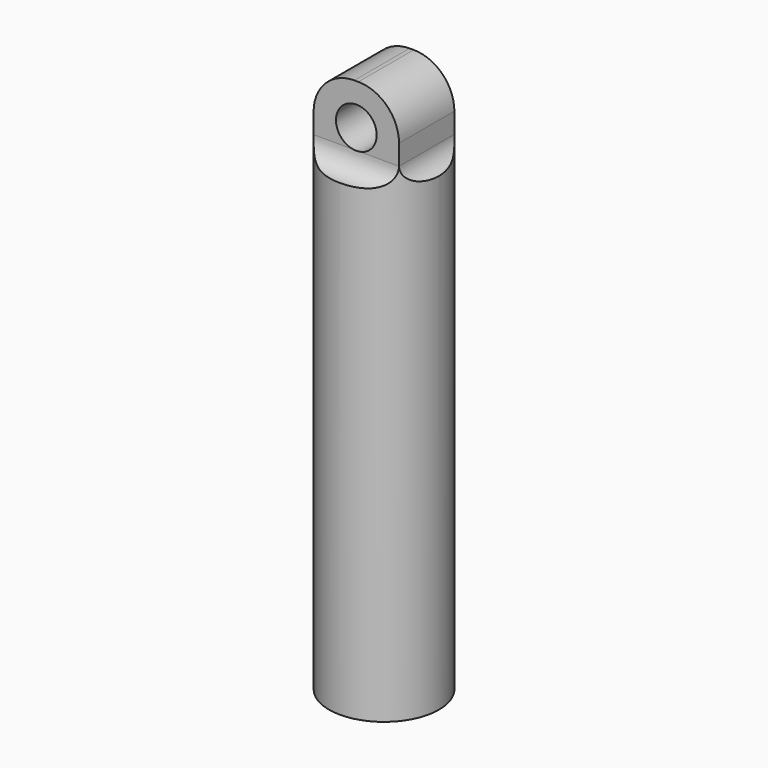
from build123d import *

# Parameters (mm, degrees)
F0_R         = 13.5
F1_DEPTH     = 115
F2_W         = 20.9761769634
F2_H         = 17
F3_DEPTH     = 20
F4_R         = 5
F5_DEPTH     = 25
F6_R         = 10
F7_T4_DEPTH  = 20.9761769634
F7_S5_R      = 5
F7_T6_DEPTH  = 13
F7_S7_R      = 13.5
F7_T8_DEPTH  = 13
F7_T12_DEPTH = 20.9761769634
F7_S13_R     = 13.5
F7_T14_DEPTH = 13
F7_S15_R     = 5
F7_T16_DEPTH = 13
F8_T4_DEPTH  = 42
F8_S5_R      = 13.5
F8_T6_DEPTH  = 23
F8_T10_DEPTH = 42
F8_S11_R     = 13.5
F8_T12_DEPTH = 23


# Not quite as in the source:
# - a fillet or chamfer that OpenCascade refuses, or shapes differently, is made with other operations: its cross-section is extruded or revolved along the edge and cut away or added


with BuildPart() as f1:
    # F0 (on Top) → F1 (new body)
    with BuildSketch(Plane.XY):
        Circle(F0_R)
    extrude(amount=F1_DEPTH)

    # F2 (on face) → F3 (join)
    with BuildSketch(Plane.XY.offset(115)):
        Rectangle(F2_W, F2_H)
    extrude(amount=F3_DEPTH)

    # F4 (on face) → F5 (cut)
    with BuildSketch(Plane.XZ.offset(8.5)):
        with Locations((0, 124.938569963)):
            Circle(F4_R)
    extrude(amount=-F5_DEPTH, mode=Mode.SUBTRACT)

    # F6
    f6_edges = [f1.edges().sort_by_distance(p)[0] for p in [
        (10.488088, 0, 135),
        (-10.488088, 0, 135),
    ]]
    fillet(f6_edges, radius=F6_R)

    # F7: fillet of radius 5 on 2 edges, made by hand


with BuildPart() as f7_tool2:
    # F7_s3 → F7_t4 (new body)
    with BuildSketch(Plane.YZ.offset(-10.4880884817)):
        with BuildLine():
            ThreePointArc((-8.5, 120), (-9.9644660941, 116.4644660941), (-13.5, 115))
            Line((-13.5, 115), (-8.5, 115))
            Line((-8.5, 115), (-8.5, 120))
        make_face()
    extrude(amount=F7_T4_DEPTH)

    # F7_s5 → F7_t6 (cut, symmetric)
    with BuildSketch(Plane.XZ.offset(11)):
        with Locations((0, 124.938569963)):
            Circle(F7_S5_R)
    extrude(amount=F7_T6_DEPTH, both=True, mode=Mode.SUBTRACT)

    # F7_s7 → F7_t8 (intersect, symmetric)
    with BuildSketch(Plane.XY.offset(117.5)):
        Circle(F7_S7_R)
    extrude(amount=F7_T8_DEPTH, both=True, mode=Mode.INTERSECT)


with BuildPart() as f1_1:
    add(f1.part)

    # F7_t1: union F7_tool2
    add(f7_tool2.part)


with BuildPart() as f7_tool10:
    # F7_s11 → F7_t12 (new body)
    with BuildSketch(Plane.YZ.offset(10.4880884817)):
        with BuildLine():
            ThreePointArc((8.5, 120), (9.9644660941, 116.4644660941), (13.5, 115))
            Line((13.5, 115), (8.5, 115))
            Line((8.5, 115), (8.5, 120))
        make_face()
    extrude(amount=-F7_T12_DEPTH)

    # F7_s13 → F7_t14 (intersect, symmetric)
    with BuildSketch(Plane.XY.offset(117.5)):
        Circle(F7_S13_R)
    extrude(amount=F7_T14_DEPTH, both=True, mode=Mode.INTERSECT)

    # F7_s15 → F7_t16 (cut, symmetric)
    with BuildSketch(Plane.XZ.offset(-11)):
        with Locations((0, 124.938569963)):
            Circle(F7_S15_R)
    extrude(amount=F7_T16_DEPTH, both=True, mode=Mode.SUBTRACT)


with BuildPart() as f1_2:
    add(f1_1.part)

    # F7_t9: union F7_tool10
    add(f7_tool10.part)

    # F8: fillet of radius 5 on 2 edges, made by hand


with BuildPart() as f8_tool2:
    # F8_s3 → F8_t4 (new body)
    with BuildSketch(Plane.XZ.offset(21)):
        with BuildLine():
            ThreePointArc((10.4880884817, 120), (11.9525545758, 116.4644660941), (15.4880884817, 115))
            Line((15.4880884817, 115), (10.4880884817, 115))
            Line((10.4880884817, 115), (10.4880884817, 120))
        make_face()
    extrude(amount=-F8_T4_DEPTH)

    # F8_s5 → F8_t6 (intersect, symmetric)
    with BuildSketch(Plane.XY.offset(117.5)):
        Circle(F8_S5_R)
    extrude(amount=F8_T6_DEPTH, both=True, mode=Mode.INTERSECT)


with BuildPart() as f1_3:
    add(f1_2.part)

    # F8_t1: union F8_tool2
    add(f8_tool2.part)


with BuildPart() as f8_tool8:
    # F8_s9 → F8_t10 (new body)
    with BuildSketch(Plane.XZ.offset(-21)):
        with BuildLine():
            ThreePointArc((-15.4880884817, 115), (-11.9525545758, 116.4644660941), (-10.4880884817, 120))
            Line((-10.4880884817, 120), (-10.4880884817, 115))
            Line((-10.4880884817, 115), (-15.4880884817, 115))
        make_face()
    extrude(amount=F8_T10_DEPTH)

    # F8_s11 → F8_t12 (intersect, symmetric)
    with BuildSketch(Plane.XY.offset(117.5)):
        Circle(F8_S11_R)
    extrude(amount=F8_T12_DEPTH, both=True, mode=Mode.INTERSECT)


with BuildPart() as f1_4:
    add(f1_3.part)

    # F8_t7: union F8_tool8
    add(f8_tool8.part)


solid = f1_4.part
